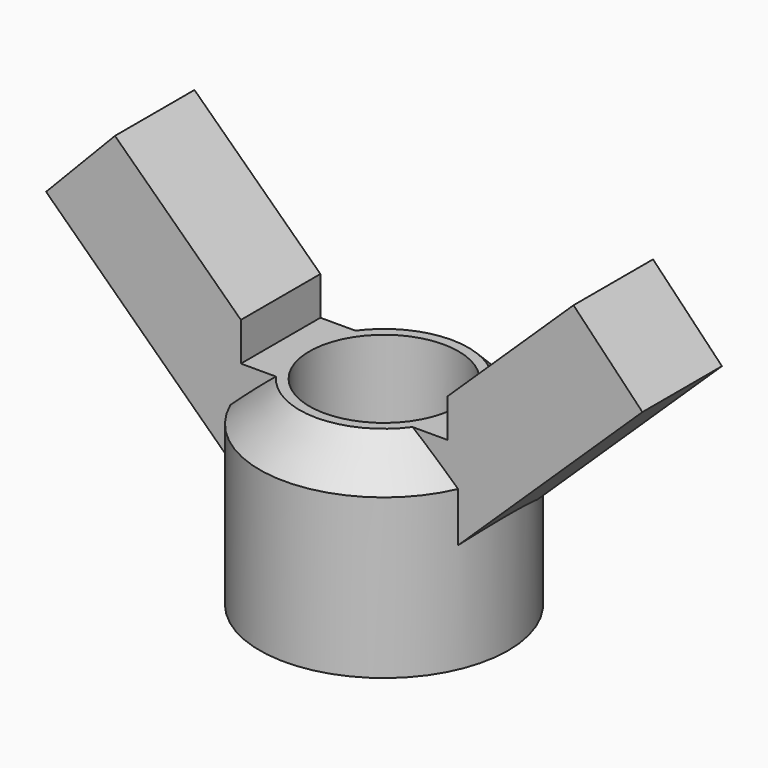
from build123d import *

# Parameters (mm, degrees)
F1_DEPTH      = 3.175
F1_DEPTH_BACK = 3.175
F2_R          = 7.9375
F2_R_2        = 4.7625
F3_DEPTH      = 12.7
F4_T4_ANGLE   = 227.2280154593
F4_T9_ANGLE   = 227.2280154593


# Not quite as in the source:
# - a fillet or chamfer that OpenCascade refuses, or shapes differently, is made with other operations: its cross-section is extruded or revolved along the edge and cut away or added


with BuildPart() as f1:
    # F0 (on Front) → F1 (new body, two sides)
    with BuildSketch(Plane.XZ) as f1_sk:
        Polygon((-19.05, 18.3173076923), (-6.604, 6.35), (-6.604, 15.1592518354), (-14.6487596518, 22.8945976544), align=None)
    extrude(amount=F1_DEPTH)
    extrude(f1_sk.sketch, amount=-F1_DEPTH_BACK)



with BuildPart() as f1b:
    # F0 (on Front) → F1, piece 2 (new body, two sides)
    with BuildSketch(Plane.XZ) as f1_2_sk:
        Polygon((6.604, 15.1592518354), (6.604, 6.35), (19.05, 18.3173076923), (14.6487596518, 22.8945976544), align=None)
    extrude(amount=F1_DEPTH)
    extrude(f1_2_sk.sketch, amount=-F1_DEPTH_BACK)


with BuildPart() as f1_1:
    add(f1.part)

    add(f1b.part)  # F3 merges F1b
    # F2 (on Top) → F3 (join)
    with BuildSketch(Plane.XY):
        Circle(F2_R)
        Circle(F2_R_2, mode=Mode.SUBTRACT)
    extrude(amount=F3_DEPTH)

    # F4: chamfer of 2.54 on 2 edges, made by hand


with BuildPart() as f4_tool2:
    # F4_s3 → F4_t4 (revolve)
    with BuildSketch(Plane(origin=(0, 0, 0), x_dir=(0, 0, 1), z_dir=(0.4005730539, 0.9162648244, 0))):
        with BuildLine():
            Line((10.088157951, -8.009342049), (12.771842049, -5.325657951))
            Line((12.771842049, -5.325657951), (12.822642049, -5.325657951))
            ThreePointArc((12.822642049, -5.325657951), (12.7508, -6.6315789755), (12.7508, -7.9375))
            Line((12.7508, -7.9375), (12.7, -7.9883))
            ThreePointArc((12.7, -7.9883), (11.3940789755, -7.9883), (10.088157951, -8.060142049))
            Line((10.088157951, -8.060142049), (10.088157951, -8.009342049))
        make_face()
    revolve(axis=Axis((0, 0, 12.7), (0, 0, 1)), revolution_arc=F4_T4_ANGLE)

    split(bisect_by=Plane.XZ.offset(3.175), keep=Keep.TOP)


with BuildPart() as f1_2:
    add(f1_1.part)

    # F4_t1: cut F4_tool2
    add(f4_tool2.part, mode=Mode.SUBTRACT)


with BuildPart() as f4_tool7:
    # F4_s8 → F4_t9 (revolve)
    with BuildSketch(Plane(origin=(0, 0, 0), x_dir=(0, 0, 1), z_dir=(-0.4005730539, -0.9162648244, 0))):
        with BuildLine():
            Line((10.088157951, -8.009342049), (12.771842049, -5.325657951))
            Line((12.771842049, -5.325657951), (12.822642049, -5.325657951))
            ThreePointArc((12.822642049, -5.325657951), (12.7508, -6.6315789755), (12.7508, -7.9375))
            Line((12.7508, -7.9375), (12.7, -7.9883))
            ThreePointArc((12.7, -7.9883), (11.3940789755, -7.9883), (10.088157951, -8.060142049))
            Line((10.088157951, -8.060142049), (10.088157951, -8.009342049))
        make_face()
    revolve(axis=Axis((0, 0, 12.7), (0, 0, 1)), revolution_arc=F4_T9_ANGLE)

    split(bisect_by=Plane.XZ.offset(-3.175), keep=Keep.BOTTOM)


with BuildPart() as f1_3:
    add(f1_2.part)

    # F4_t6: cut F4_tool7
    add(f4_tool7.part, mode=Mode.SUBTRACT)


solid = f1_3.part
